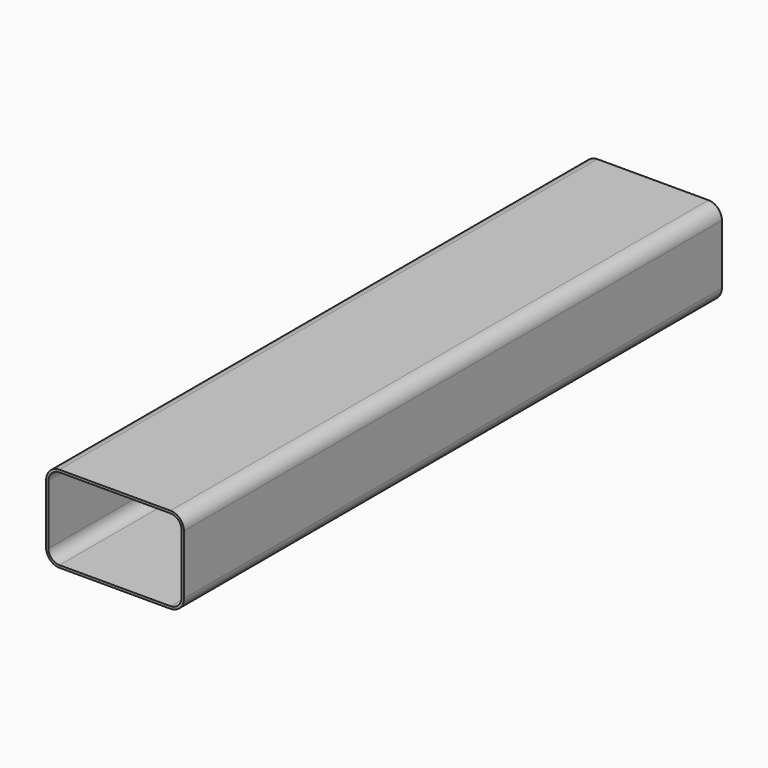
from build123d import *

# Parameters (mm, degrees)
F1_DEPTH = 300


# Not quite as in the source:
# - a pattern or mirror of a feature is missing from the dataset's text; its kind, count and spacing are read off the source's solid


with BuildPart() as f1:
    # F0 (on Front) → F1 (new body)
    with BuildSketch(Plane.XZ):
        with BuildLine():
            ThreePointArc((51.25, 22.125), (48.3210678119, 29.1960678119), (41.25, 32.125))
            Line((41.25, 32.125), (-41.25, 32.125))
            ThreePointArc((-41.25, 32.125), (-48.3210678119, 29.1960678119), (-51.25, 22.125))
            Line((-51.25, 22.125), (-51.25, -22.125))
            ThreePointArc((-51.25, -22.125), (-48.3210678119, -29.1960678119), (-41.25, -32.125))
            Line((-41.25, -32.125), (41.25, -32.125))
            ThreePointArc((41.25, -32.125), (48.3210678119, -29.1960678119), (51.25, -22.125))
            Line((51.25, -22.125), (51.25, 22.125))
        make_face()
        with BuildLine():
            Line((-49.5, -22.125), (-49.5, 22.125))
            ThreePointArc((-49.5, 22.125), (-47.0836309448, 27.9586309448), (-41.25, 30.375))
            Line((-41.25, 30.375), (41.25, 30.375))
            ThreePointArc((41.25, 30.375), (47.0836309448, 27.9586309448), (49.5, 22.125))
            Line((49.5, 22.125), (49.5, -22.125))
            ThreePointArc((49.5, -22.125), (47.0836309448, -27.9586309448), (41.25, -30.375))
            Line((41.25, -30.375), (-41.25, -30.375))
            ThreePointArc((-41.25, -30.375), (-47.0836309448, -27.9586309448), (-49.5, -22.125))
        make_face(mode=Mode.SUBTRACT)
    extrude(amount=-F1_DEPTH)

    # F1_copies: F1 across plane


with BuildPart() as f1_1:
    add(f1.part)
    add(f1.part.mirror(Plane.ZX.offset(250)))


solid = f1_1.part
